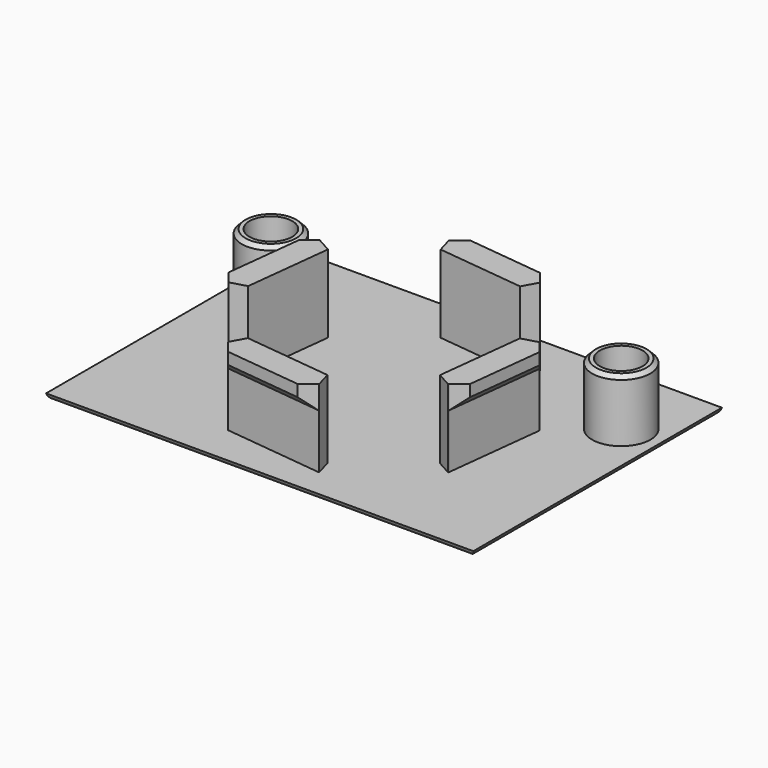
from build123d import *

# Parameters (mm, degrees)
F0_W         = 55
F0_H         = 40
F1_DEPTH     = 0.8
F3_DEPTH     = 10
F2_R         = 3.75
F2_R_2       = 2.75
F4_DEPTH     = 8
F5_SIZE      = 0.5
F6_W         = 12.8945924119
F6_H         = 3
F7_DEPTH     = 1.5
F8_SIZE      = 1.49999
F9_SIZE      = 1.49999
F10_W        = 12.8768104754
F10_H        = 3
F11_DEPTH    = 1.5
F12_SIZE     = 1.49999
F13_W        = 12.9808257885
F13_H        = 3
F14_DEPTH    = 1.5
F15_SIZE     = 1.49999
F16_W        = 12.9808257885
F16_H        = 3
F17_DEPTH    = 1.5
F18_SIZE     = 1.49999
F19_T1_DEPTH = 59.8989794856
F19_T3_DEPTH = 44.8989794856


# Not quite as in the source:
# - a fillet or chamfer that OpenCascade refuses, or shapes differently, is made with other operations: its cross-section is extruded or revolved along the edge and cut away or added
# - a fillet or chamfer is up to 0.001 mm smaller than in the source, because OpenCascade refuses the exact size


with BuildPart() as f1:
    # F0 (on Top) → F1 (new body)
    with BuildSketch(Plane.XY):
        Rectangle(F0_W, F0_H)
    extrude(amount=F1_DEPTH)

    # F2 (on face) → F3 (join)
    with BuildSketch(Plane.XY.offset(0.8)):
        Polygon((7.1650690396, 12.9448085418), (8.2134181145, 14.8388137473), (-4.68486218, 16.3003894709), (-4.0868929955, 14.2198308067), align=None)
        with BuildLine():
            Line((-8.2134181145, -14.8388137473), (4.5991771643, -16.2906800263))
            ThreePointArc((4.5991771643, -16.2906800263), (4.6374749925, -16.2797221091), (4.6757470388, -16.268674482))
            Line((4.6757470388, -16.268674482), (4.0868929955, -14.2198308067))
            Line((4.0868929955, -14.2198308067), (-7.1650690396, -12.9448085418))
            Line((-7.1650690396, -12.9448085418), (-8.2134181145, -14.8388137473))
        make_face()
        Polygon((-14.8388137473, 8.2134181145), (-16.3003894709, -4.68486218), (-14.2198308067, -4.0868929955), (-12.9448085418, 7.1650690396), align=None)
        with BuildLine():
            Line((14.8505253486, -8.1100642381), (16.3003894709, 4.68486218))
            Line((16.3003894709, 4.68486218), (14.2198308067, 4.0868929955))
            Line((14.2198308067, 4.0868929955), (12.9448085418, -7.1650690396))
            Line((12.9448085418, -7.1650690396), (14.8041096105, -8.1942090597))
            ThreePointArc((14.8041096105, -8.1942090597), (14.8273769365, -8.1521694464), (14.8505253486, -8.1100642381))
        make_face()
    extrude(amount=F3_DEPTH)

    # F2 (on face) → F4 (join)
    with BuildSketch(Plane.XY.offset(0.8)):
        with Locations((22.4918836008, 10.0589259832)):
            Circle(F2_R)
        with Locations((22.4918836008, 10.0589259832)):
            Circle(F2_R_2, mode=Mode.SUBTRACT)
        with Locations((-22.6081163992, 10.0589259832)):
            Circle(F2_R)
        with Locations((-22.6081163992, 10.0589259832)):
            Circle(F2_R_2, mode=Mode.SUBTRACT)
    extrude(amount=F4_DEPTH)

    # F5
    f5_edges = [f1.edges().sort_by_distance(p)[0] for p in [
        (-26.358116, 10.058926, 8.8),
        (18.741884, 10.058926, 8.8),
    ]]
    chamfer(f5_edges, length=F5_SIZE)

    # F6 (on face) → F7 (join)
    with BuildSketch(Plane(origin=(-1.7642779672, -15.5696016091, 0), x_dir=(0.9936409674, -0.1125949726, 0), z_dir=(-0.1125949726, -0.9936409674, 0))):
        with Locations((-0.0431166883, 9.3)):
            Rectangle(F6_W, F6_H)
    extrude(amount=F7_DEPTH)

    # F8 (size 1.5 in the source; OpenCascade refuses exactly that, so slightly less here)
    f8_edges = [f1.edges().sort_by_distance(p)[0] for p in [
        (-1.976013, -17.055208, 7.8),
    ]]
    chamfer(f8_edges, length=F8_SIZE)

    # F9 (size 1.5 in the source; OpenCascade refuses exactly that, so slightly less here)
    f9_edges = [f1.edges().sort_by_distance(p)[0] for p in [
        (-8.382311, -16.329275, 10.049995),
        (4.430285, -17.781141, 10.049995),
    ]]
    chamfer(f9_edges, length=F9_SIZE)

    # F10 (on face) → F11 (join)
    with BuildSketch(Plane(origin=(15.5696016091, -1.7642779672, 0), x_dir=(0.1125949726, 0.9936409674, 0), z_dir=(0.9936409674, -0.1125949726, 0))):
        with Locations((0.0520076565, 9.3)):
            Rectangle(F10_W, F10_H)
    extrude(amount=F11_DEPTH)

    # F12 (size 1.5 in the source; OpenCascade refuses exactly that, so slightly less here)
    f12_edges = [f1.edges().sort_by_distance(p)[0] for p in [
        (17.065919, -1.881493, 7.8),
        (16.340987, -8.278957, 9.3),
        (17.790851, 4.51597, 9.3),
    ]]
    chamfer(f12_edges, length=F12_SIZE)

    # F13 (on face) → F14 (join)
    with BuildSketch(Plane(origin=(1.7642779672, 15.5696016091, 0), x_dir=(-0.9936409674, 0.1125949726, 0), z_dir=(0.1125949726, 0.9936409674, 0))):
        with Locations((0, 9.3)):
            Rectangle(F13_W, F13_H)
    extrude(amount=F14_DEPTH)

    # F15 (size 1.5 in the source; OpenCascade refuses exactly that, so slightly less here)
    f15_edges = [f1.edges().sort_by_distance(p)[0] for p in [
        (8.382311, 16.329275, 9.3),
        (1.93317, 17.060063, 7.8),
        (-4.51597, 17.790851, 9.3),
    ]]
    chamfer(f15_edges, length=F15_SIZE)

    # F16 (on face) → F17 (join)
    with BuildSketch(Plane(origin=(-15.5696016091, 1.7642779672, 0), x_dir=(-0.1125949726, -0.9936409674, 0), z_dir=(-0.9936409674, 0.1125949726, 0))):
        with Locations((0, 9.3)):
            Rectangle(F16_W, F16_H)
    extrude(amount=F17_DEPTH)

    # F18 (size 1.5 in the source; OpenCascade refuses exactly that, so slightly less here)
    f18_edges = [f1.edges().sort_by_distance(p)[0] for p in [
        (-16.329275, 8.382311, 9.3),
        (-17.060063, 1.93317, 7.8),
        (-17.790851, -4.51597, 9.3),
    ]]
    chamfer(f18_edges, length=F18_SIZE)

    # F19: fillet of radius 1 on 4 edges, made by hand

    # F19_s2 → F19_t1 (cut)
    with BuildSketch(Plane.YZ.offset(-29.9494897428)):
        with BuildLine():
            ThreePointArc((-20, 0.8), (-19.6526596349, 0.2254033308), (-19.0202041029, 0))
            Line((-19.0202041029, 0), (-20, 0))
            Line((-20, 0), (-20, 0.8))
        make_face()
        with BuildLine():
            ThreePointArc((20, 0.8), (19.6526596349, 0.2254033308), (19.0202041029, 0))
            Line((19.0202041029, 0), (20, 0))
            Line((20, 0), (20, 0.8))
        make_face()
    extrude(amount=F19_T1_DEPTH, mode=Mode.SUBTRACT)

    # F19_s4 → F19_t3 (cut)
    with BuildSketch(Plane.XZ.offset(-22.4494897428)):
        with BuildLine():
            ThreePointArc((27.5, 0.8), (27.1526596349, 0.2254033308), (26.5202041029, 0))
            Line((26.5202041029, 0), (27.5, 0))
            Line((27.5, 0), (27.5, 0.8))
        make_face()
        with BuildLine():
            ThreePointArc((-27.5, 0.8), (-27.1526596349, 0.2254033308), (-26.5202041029, 0))
            Line((-26.5202041029, 0), (-27.5, 0))
            Line((-27.5, 0), (-27.5, 0.8))
        make_face()
    extrude(amount=F19_T3_DEPTH, mode=Mode.SUBTRACT)


solid = f1.part
